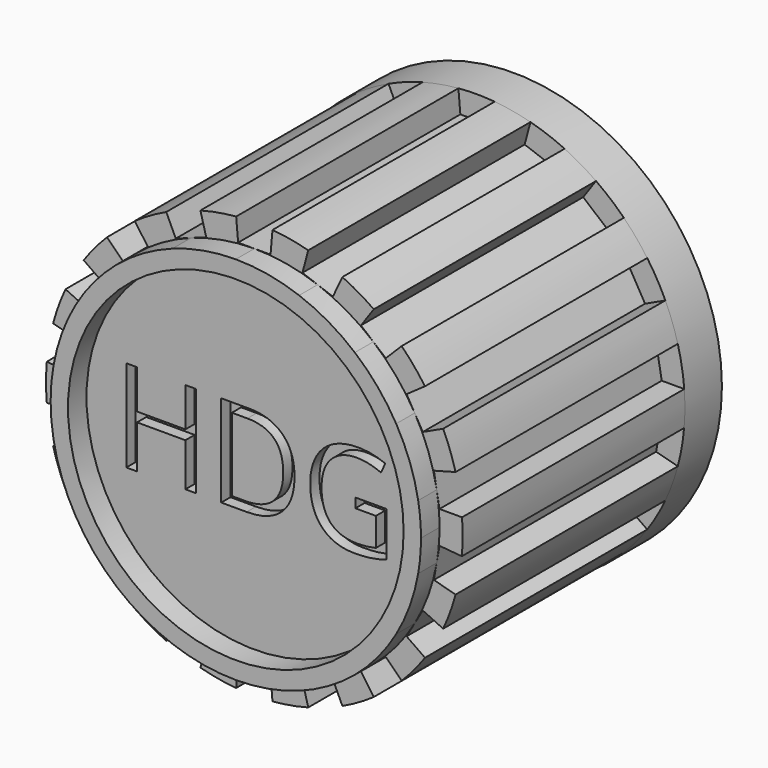
from build123d import *

# Parameters (mm, degrees)
F1_DEPTH     = 9.525
F2_R         = 7.14375
F3_DEPTH     = 1.5875
F4_R         = 5.7546875
F5_DEPTH     = 0.79375
F6_TEXT_SIZE = 4.4097222222
F7_DEPTH     = 0.396875
F8_R         = 3.571875
F9_DEPTH     = 9.525
F10_R        = 1.190625
F11_DEPTH    = 12.7


# Not quite as in the source:
# - a length typed as a fraction of an inch, garbled in the dataset ("3 / 203.2 mm" for 3/8 in), is restored
# - Text() gives the source's letters only with a copy of the font that has no kerning and outlines rounded to 1/6400 em; it was checked with that copy


with BuildPart() as f1:
    # F0 (on Front) → F1 (new body)
    with BuildSketch(Plane.XZ):
        with BuildLine():
            Line((-0.5555530134, 6.35), (-0.6226188373, 7.1165658745))
            ThreePointArc((-0.6226188373, 7.1165658745), (-1.2404991692, 7.0352203856), (-1.8489385535, 6.9003326216))
            Line((-1.8489385535, 6.9003326216), (-1.649778843, 6.1570584633))
            Line((-1.649778843, 6.1570584633), (-2.6938769773, 5.7770378207))
            Line((-2.6938769773, 5.7770378207), (-3.0190792073, 6.4744362536))
            ThreePointArc((-3.0190792073, 6.4744362536), (-3.571875, 6.1866689783), (-4.0974866672, 5.8518174164))
            Line((-4.0974866672, 5.8518174164), (-3.6561230227, 5.2214848073))
            Line((-3.6561230227, 5.2214848073), (-4.5072796203, 4.5072796203))
            Line((-4.5072796203, 4.5072796203), (-5.0513940681, 5.0513940681))
            ThreePointArc((-5.0513940681, 5.0513940681), (-5.4724299905, 4.5919139867), (-5.8518174164, 4.0974866672))
            Line((-5.8518174164, 4.0974866672), (-5.2214848073, 3.6561230227))
            Line((-5.2214848073, 3.6561230227), (-5.7770378207, 2.6938769773))
            Line((-5.7770378207, 2.6938769773), (-6.4744362536, 3.0190792073))
            ThreePointArc((-6.4744362536, 3.0190792073), (-6.7129291597, 2.4433063989), (-6.9003326216, 1.8489385535))
            Line((-6.9003326216, 1.8489385535), (-6.1570584633, 1.649778843))
            Line((-6.1570584633, 1.649778843), (-6.35, 0.5555530134))
            Line((-6.35, 0.5555530134), (-7.1165658745, 0.6226188373))
            ThreePointArc((-7.1165658745, 0.6226188373), (-7.14375, 0), (-7.1165658745, -0.6226188373))
            Line((-7.1165658745, -0.6226188373), (-6.35, -0.5555530134))
            Line((-6.35, -0.5555530134), (-6.1570584633, -1.649778843))
            Line((-6.1570584633, -1.649778843), (-6.9003326216, -1.8489385535))
            ThreePointArc((-6.9003326216, -1.8489385535), (-6.7129291597, -2.4433063989), (-6.4744362536, -3.0190792073))
            Line((-6.4744362536, -3.0190792073), (-5.7770378207, -2.6938769773))
            Line((-5.7770378207, -2.6938769773), (-5.2214848073, -3.6561230227))
            Line((-5.2214848073, -3.6561230227), (-5.8518174164, -4.0974866672))
            ThreePointArc((-5.8518174164, -4.0974866672), (-5.4724299905, -4.5919139867), (-5.0513940681, -5.0513940681))
            Line((-5.0513940681, -5.0513940681), (-4.5072796203, -4.5072796203))
            Line((-4.5072796203, -4.5072796203), (-3.6561230227, -5.2214848073))
            Line((-3.6561230227, -5.2214848073), (-4.0974866672, -5.8518174164))
            ThreePointArc((-4.0974866672, -5.8518174164), (-3.571875, -6.1866689783), (-3.0190792073, -6.4744362536))
            Line((-3.0190792073, -6.4744362536), (-2.6938769773, -5.7770378207))
            Line((-2.6938769773, -5.7770378207), (-1.649778843, -6.1570584633))
            Line((-1.649778843, -6.1570584633), (-1.8489385535, -6.9003326216))
            ThreePointArc((-1.8489385535, -6.9003326216), (-1.2404991692, -7.0352203856), (-0.6226188373, -7.1165658745))
            Line((-0.6226188373, -7.1165658745), (-0.5555530134, -6.35))
            Line((-0.5555530134, -6.35), (0.5555530134, -6.35))
            Line((0.5555530134, -6.35), (0.6226188373, -7.1165658745))
            ThreePointArc((0.6226188373, -7.1165658745), (1.2404991692, -7.0352203856), (1.8489385535, -6.9003326216))
            Line((1.8489385535, -6.9003326216), (1.649778843, -6.1570584633))
            Line((1.649778843, -6.1570584633), (2.6938769773, -5.7770378207))
            Line((2.6938769773, -5.7770378207), (3.0190792073, -6.4744362536))
            ThreePointArc((3.0190792073, -6.4744362536), (3.571875, -6.1866689783), (4.0974866672, -5.8518174164))
            Line((4.0974866672, -5.8518174164), (3.6561230227, -5.2214848073))
            Line((3.6561230227, -5.2214848073), (4.5072796203, -4.5072796203))
            Line((4.5072796203, -4.5072796203), (5.0513940681, -5.0513940681))
            ThreePointArc((5.0513940681, -5.0513940681), (5.4724299905, -4.5919139867), (5.8518174164, -4.0974866672))
            Line((5.8518174164, -4.0974866672), (5.2214848073, -3.6561230227))
            Line((5.2214848073, -3.6561230227), (5.7770378207, -2.6938769773))
            Line((5.7770378207, -2.6938769773), (6.4744362536, -3.0190792073))
            ThreePointArc((6.4744362536, -3.0190792073), (6.7129291597, -2.4433063989), (6.9003326216, -1.8489385535))
            Line((6.9003326216, -1.8489385535), (6.1570584633, -1.649778843))
            Line((6.1570584633, -1.649778843), (6.35, -0.5555530134))
            Line((6.35, -0.5555530134), (7.1165658745, -0.6226188373))
            ThreePointArc((7.1165658745, -0.6226188373), (7.1436707586, -0.0336475101), (7.1221151993, 0.5555530134))
            Line((7.1221151993, 0.5555530134), (6.35, 0.5555530134))
            Line((6.35, 0.5555530134), (6.1570584633, 1.649778843))
            Line((6.1570584633, 1.649778843), (6.9003326216, 1.8489385535))
            ThreePointArc((6.9003326216, 1.8489385535), (6.7129291597, 2.4433063989), (6.4744362536, 3.0190792073))
            Line((6.4744362536, 3.0190792073), (5.7770378207, 2.6938769773))
            Line((5.7770378207, 2.6938769773), (5.2214848073, 3.6561230227))
            Line((5.2214848073, 3.6561230227), (5.8518174164, 4.0974866672))
            ThreePointArc((5.8518174164, 4.0974866672), (5.4724299905, 4.5919139867), (5.0513940681, 5.0513940681))
            Line((5.0513940681, 5.0513940681), (4.5072796203, 4.5072796203))
            Line((4.5072796203, 4.5072796203), (3.6561230227, 5.2214848073))
            Line((3.6561230227, 5.2214848073), (4.0974866672, 5.8518174164))
            ThreePointArc((4.0974866672, 5.8518174164), (3.571875, 6.1866689783), (3.0190792073, 6.4744362536))
            Line((3.0190792073, 6.4744362536), (2.6938769773, 5.7770378207))
            Line((2.6938769773, 5.7770378207), (1.649778843, 6.1570584633))
            Line((1.649778843, 6.1570584633), (1.8489385535, 6.9003326216))
            ThreePointArc((1.8489385535, 6.9003326216), (1.2404991692, 7.0352203856), (0.6226188373, 7.1165658745))
            Line((0.6226188373, 7.1165658745), (0.5555530134, 6.35))
            Line((0.5555530134, 6.35), (-0.5555530134, 6.35))
        make_face()
    extrude(amount=F1_DEPTH)

    # F2 (on face) → F3 (join)
    with BuildSketch(Plane(origin=(0, 0, 0), x_dir=(-1, 0, 0), z_dir=(0, 1, 0))):
        Circle(F2_R)
    extrude(amount=F3_DEPTH)

    # F4 (on face) → F5 (join)
    with BuildSketch(Plane.XZ.offset(9.525)):
        with BuildLine():
            ThreePointArc((6.2535294448, -1.1026647193), (6.3258363864, -0.553438355), (6.35, 0))
            ThreePointArc((6.35, 0), (6.3258363886, 0.5534383295), (6.2535294537, 1.1026646688))
            ThreePointArc((6.2535294537, 1.1026646688), (5.9670483798, 2.1718272567), (5.49926137, 3.1749999031))
            ThreePointArc((5.49926137, 3.1749999031), (4.8643822541, 4.0817012735), (4.0817013319, 4.8643822051))
            ThreePointArc((4.0817013319, 4.8643822051), (3.174999958, 5.4992613383), (2.1718278063, 5.9670481798))
            ThreePointArc((2.1718278063, 5.9670481798), (1.1026658738, 6.2535292412), (0, 6.35))
            ThreePointArc((0, 6.35), (-1.1026658738, 6.2535292412), (-2.1718278063, 5.9670481798))
            ThreePointArc((-2.1718278063, 5.9670481798), (-3.174999958, 5.4992613383), (-4.0817013319, 4.8643822051))
            ThreePointArc((-4.0817013319, 4.8643822051), (-4.8643822183, 4.0817013161), (-5.4992613143, 3.1749999996))
            ThreePointArc((-5.4992613143, 3.1749999996), (-5.9670483513, 2.171827335), (-6.2535294441, 1.1026647232))
            ThreePointArc((-6.2535294441, 1.1026647232), (-6.35, -2e-10), (-6.253529444, -1.1026647236))
            ThreePointArc((-6.253529444, -1.1026647236), (-5.9670483512, -2.1718273352), (-5.4992613143, -3.1749999996))
            ThreePointArc((-5.4992613143, -3.1749999996), (-4.8643822183, -4.0817013161), (-4.0817013319, -4.8643822051))
            ThreePointArc((-4.0817013319, -4.8643822051), (-3.1750000369, -5.4992612927), (-2.1718279774, -5.9670481175))
            ThreePointArc((-2.1718279774, -5.9670481175), (-1.1026659635, -6.2535292254), (0, -6.35))
            ThreePointArc((0, -6.35), (1.1026659161, -6.2535292338), (2.1718278871, -5.9670481504))
            ThreePointArc((2.1718278871, -5.9670481504), (3.1749999655, -5.499261334), (4.0817012792, -4.8643822493))
            ThreePointArc((4.0817012792, -4.8643822493), (4.8643821773, -4.081701365), (5.4992612849, -3.1750000505))
            ThreePointArc((5.4992612849, -3.1750000505), (5.9670483419, -2.1718273608), (6.2535294448, -1.1026647193))
        make_face()
        Circle(F4_R, mode=Mode.SUBTRACT)
    extrude(amount=F5_DEPTH)

    # F6 (on face) → F7 (cut)
    with BuildSketch(Plane.XZ.offset(9.525)):
        with Locations((-4.8210666233, -1.6845211491)):
            Text('HDG', F6_TEXT_SIZE, font='Open Sans', text_align=(TextAlign.LEFT, TextAlign.BOTTOM))
    extrude(amount=-F7_DEPTH, mode=Mode.SUBTRACT)

    # F8 (on face) → F9 (cut)
    with BuildSketch(Plane(origin=(0, 1.5875, 0), x_dir=(-1, 0, 0), z_dir=(0, 1, 0))):
        Circle(F8_R)
    extrude(amount=-F9_DEPTH, mode=Mode.SUBTRACT)

    # F10 (on Right) → F11 (cut)
    with BuildSketch(Plane.YZ):
        with Locations((-0.8031820762, 0)):
            Circle(F10_R)
    extrude(amount=-F11_DEPTH, mode=Mode.SUBTRACT)


solid = f1.part
